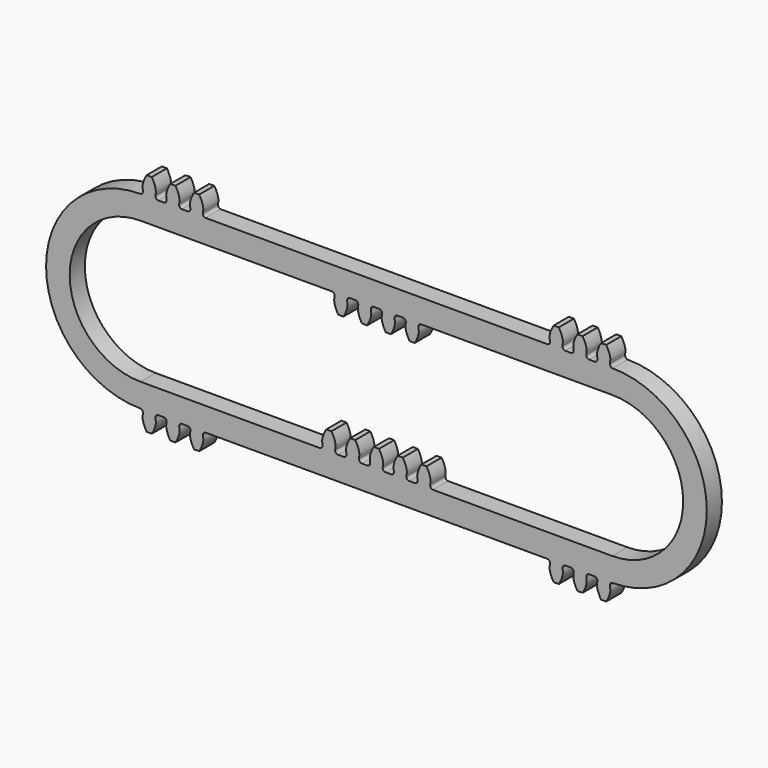
from build123d import *

# Parameters (mm, degrees)
F1_DEPTH = 5.08


# Not quite as in the source:
# - ends of sketch curves that miss each other by under 0.0002 mm in the source are joined
# - the dataset's text gives a spline's control points without its knots; the knots are read off the source's solid


with BuildPart() as f1:
    # F0 (on Front) → F1 (new body)
    with BuildSketch(Plane.XZ):
        with BuildLine():
            ThreePointArc((-63.3810963483, 25.3901347093), (-63.3753119036, 25.3901346444), (-63.3695274591, 25.3901332617))
            Line((-63.3695274591, 25.3901332617), (-58.7276592851, 25.3901332617))
            ThreePointArc((-58.7276592851, 25.3901332617), (-59.218266422, 25.7011127201), (-59.3684714986, 26.2622205719))
            add(Edge.make_bspline(
                [(-59.3684714986, 26.2622205719), (-59.31250661, 26.6931994762), (-59.2566199012, 27.1335892143), (-59.2570794401, 27.1878744736), (-59.2556284349, 27.2924728418), (-59.2623142438, 27.4188463575), (-59.2785741325, 27.5871922152), (-59.3088462635, 27.7897160279), (-59.3564984328, 28.027587018), (-59.4251457106, 28.298787), (-59.5181989128, 28.6019292415), (-59.6390373643, 28.9351012863), (-59.7906998965, 29.2962093017), (-59.9768979086, 29.6829308745), (-60.1697133275, 30.040270436), (-60.3087276421, 30.2685072323), (-60.3647969547, 30.359069462)],
                knots=[0.0609120431, 0.0609120431, 0.0609120431, 0.0609120431, 0.1648778545, 0.1947232852, 0.233253523, 0.2788430996, 0.3305368133, 0.38768636, 0.4498144648, 0.5165507531, 0.587596956, 0.6627061681, 0.7416696063, 0.8243077052, 0.9104638785, 0.9670212386, 0.9670212386, 0.9670212386, 0.9670212386], degree=3))
            Line((-60.3647969547, 30.359069462), (-61.7439586786, 30.359069462))
            add(Edge.make_bspline(
                [(-62.7402841346, 26.2622205719), (-62.7962490233, 26.6931994762), (-62.8521357321, 27.1335892143), (-62.8516761931, 27.1878744736), (-62.8531271984, 27.2924728418), (-62.8464413895, 27.4188463575), (-62.8301815007, 27.5871922152), (-62.7999093697, 27.7897160279), (-62.7522572004, 28.027587018), (-62.6836099226, 28.298787), (-62.5905567204, 28.6019292415), (-62.4697182689, 28.9351012863), (-62.3180557368, 29.2962093017), (-62.1318577246, 29.6829308745), (-61.9390423057, 30.040270436), (-61.8000279911, 30.2685072323), (-61.7439586786, 30.359069462)],
                knots=[0.0609120431, 0.0609120431, 0.0609120431, 0.0609120431, 0.1648778545, 0.1947232852, 0.233253523, 0.2788430996, 0.3305368133, 0.38768636, 0.4498144648, 0.5165507531, 0.587596956, 0.6627061681, 0.7416696063, 0.8243077052, 0.9104638785, 0.9670212386, 0.9670212386, 0.9670212386, 0.9670212386], degree=3))
            ThreePointArc((-62.7402841346, 26.2622205719), (-62.8904892112, 25.7011127201), (-63.3810963483, 25.3901347093))
        make_face()
        with BuildLine():
            Line((-58.7276592851, 25.3901332617), (-63.3695274591, 25.3901332617))
            ThreePointArc((-63.3695274591, 25.3901332617), (-63.3753119036, 25.3901346444), (-63.3810963483, 25.3901347093))
            ThreePointArc((-63.3810963483, 25.3901347093), (-88.7686237693, 0), (-63.3810963483, -25.3901347093))
            ThreePointArc((-63.3810963483, -25.3901347093), (-63.3753119036, -25.3901346444), (-63.3695274591, -25.3901332617))
            Line((-63.3695274591, -25.3901332617), (-58.7276592851, -25.3901332617))
            Line((-58.7276592851, -25.3901332617), (-57.0234432817, -25.3901332617))
            Line((-57.0234432817, -25.3901332617), (-52.3700062186, -25.3901332617))
            Line((-52.3700062186, -25.3901332617), (-50.6370496005, -25.3901332617))
            Line((-50.6370496005, -25.3901332617), (-45.9836125374, -25.3901332617))
            Line((-45.9836125374, -25.3901332617), (45.9836125374, -25.3901332617))
            Line((45.9836125374, -25.3901332617), (50.6370496005, -25.3901332617))
            Line((50.6370496005, -25.3901332617), (52.3700062186, -25.3901332617))
            Line((52.3700062186, -25.3901332617), (57.0234432817, -25.3901332617))
            Line((57.0234432817, -25.3901332617), (58.7276592851, -25.3901332617))
            Line((58.7276592851, -25.3901332617), (63.3695274591, -25.3901332617))
            ThreePointArc((63.3695274591, -25.3901332617), (63.3753119036, -25.3901346444), (63.3810963483, -25.3901347093))
            ThreePointArc((63.3810963483, -25.3901347093), (88.7686237693, 0), (63.3810963483, 25.3901347093))
            ThreePointArc((63.3810963483, 25.3901347093), (63.3753119036, 25.3901346444), (63.3695274591, 25.3901332617))
            Line((63.3695274591, 25.3901332617), (58.7276592851, 25.3901332617))
            Line((58.7276592851, 25.3901332617), (57.0234432817, 25.3901332617))
            Line((57.0234432817, 25.3901332617), (52.3700062186, 25.3901332617))
            Line((52.3700062186, 25.3901332617), (50.6370496005, 25.3901332617))
            Line((50.6370496005, 25.3901332617), (45.9836125374, 25.3901332617))
            Line((45.9836125374, 25.3901332617), (-45.9836125374, 25.3901332617))
            Line((-45.9836125374, 25.3901332617), (-50.6370496005, 25.3901332617))
            Line((-50.6370496005, 25.3901332617), (-52.3700062186, 25.3901332617))
            Line((-52.3700062186, 25.3901332617), (-57.0234432817, 25.3901332617))
            Line((-57.0234432817, 25.3901332617), (-58.7276592851, 25.3901332617))
        make_face()
        with BuildLine():
            ThreePointArc((-1.685906318, -18.1751586497), (-1.8361113946, -18.7362665015), (-2.3267185315, -19.0472459599))
            Line((-2.3267185315, -19.0472459599), (-4.0499982424, -19.0472459599))
            ThreePointArc((-4.0499982424, -19.0472459599), (-4.5406053793, -18.7362665015), (-4.6908104559, -18.1751586497))
            add(Edge.make_bspline(
                [(-4.6908104559, -18.1751586497), (-4.6348455673, -17.7441797454), (-4.5789588585, -17.3037900072), (-4.5794183974, -17.2495047479), (-4.5779673922, -17.1449063798), (-4.5846532011, -17.018532864), (-4.6009130899, -16.8501870063), (-4.6311852208, -16.6476631937), (-4.6788373902, -16.4097922035), (-4.747484668, -16.1385922215), (-4.8405378702, -15.8354499801), (-4.9613763217, -15.5022779353), (-5.1130388538, -15.1411699198), (-5.299236866, -14.754448347), (-5.4920522849, -14.3971087856), (-5.6310665994, -14.1688719893), (-5.687135912, -14.0783097595)],
                knots=[0.0609120431, 0.0609120431, 0.0609120431, 0.0609120431, 0.1648778545, 0.1947232852, 0.233253523, 0.2788430996, 0.3305368133, 0.38768636, 0.4498144648, 0.5165507531, 0.587596956, 0.6627061681, 0.7416696063, 0.8243077052, 0.9104638785, 0.9670212386, 0.9670212386, 0.9670212386, 0.9670212386], degree=3))
            Line((-5.687135912, -14.0783097595), (-6.376716774, -14.0783097595))
            Line((-6.376716774, -14.0783097595), (-7.0662976359, -14.0783097595))
            add(Edge.make_bspline(
                [(-8.062623092, -18.1751586497), (-8.1185879806, -17.7441797454), (-8.1744746894, -17.3037900072), (-8.1740151505, -17.2495047479), (-8.1754661557, -17.1449063798), (-8.1687803468, -17.018532864), (-8.1525204581, -16.8501870063), (-8.1222483271, -16.6476631937), (-8.0745961578, -16.4097922035), (-8.0059488799, -16.1385922215), (-7.9128956777, -15.8354499801), (-7.7920572263, -15.5022779353), (-7.6403946941, -15.1411699198), (-7.454196682, -14.754448347), (-7.261381263, -14.3971087856), (-7.1223669485, -14.1688719893), (-7.0662976359, -14.0783097595)],
                knots=[0.0609120431, 0.0609120431, 0.0609120431, 0.0609120431, 0.1648778545, 0.1947232852, 0.233253523, 0.2788430996, 0.3305368133, 0.38768636, 0.4498144648, 0.5165507531, 0.587596956, 0.6627061681, 0.7416696063, 0.8243077052, 0.9104638785, 0.9670212386, 0.9670212386, 0.9670212386, 0.9670212386], degree=3))
            ThreePointArc((-8.062623092, -18.1751586497), (-8.2128281686, -18.7362665015), (-8.7034353055, -19.0472459599))
            Line((-8.7034353055, -19.0472459599), (-10.4555296712, -19.0472459599))
            ThreePointArc((-10.4555296712, -19.0472459599), (-10.9461368081, -18.7362665015), (-11.0963418847, -18.1751586497))
            add(Edge.make_bspline(
                [(-11.0963418847, -18.1751586497), (-11.0403769961, -17.7441797454), (-10.9844902873, -17.3037900072), (-10.9849498262, -17.2495047479), (-10.983498821, -17.1449063798), (-10.9901846299, -17.018532864), (-11.0064445186, -16.8501870063), (-11.0367166496, -16.6476631937), (-11.0843688189, -16.4097922035), (-11.1530160967, -16.1385922215), (-11.2460692989, -15.8354499801), (-11.3669077504, -15.5022779353), (-11.5185702826, -15.1411699198), (-11.7047682947, -14.754448347), (-11.8975837136, -14.3971087856), (-12.0365980282, -14.1688719893), (-12.0926673408, -14.0783097595)],
                knots=[0.0609120431, 0.0609120431, 0.0609120431, 0.0609120431, 0.1648778545, 0.1947232852, 0.233253523, 0.2788430996, 0.3305368133, 0.38768636, 0.4498144648, 0.5165507531, 0.587596956, 0.6627061681, 0.7416696063, 0.8243077052, 0.9104638785, 0.9670212386, 0.9670212386, 0.9670212386, 0.9670212386], degree=3))
            Line((-12.0926673408, -14.0783097595), (-12.7822482027, -14.0783097595))
            Line((-12.7822482027, -14.0783097595), (-13.4718290647, -14.0783097595))
            add(Edge.make_bspline(
                [(-14.4681545207, -18.1751586497), (-14.5241194093, -17.7441797454), (-14.5800061182, -17.3037900072), (-14.5795465792, -17.2495047479), (-14.5809975845, -17.1449063798), (-14.5743117756, -17.018532864), (-14.5580518868, -16.8501870063), (-14.5277797558, -16.6476631937), (-14.4801275865, -16.4097922035), (-14.4114803087, -16.1385922215), (-14.3184271065, -15.8354499801), (-14.197588655, -15.5022779353), (-14.0459261229, -15.1411699198), (-13.8597281107, -14.754448347), (-13.6669126918, -14.3971087856), (-13.5278983772, -14.1688719893), (-13.4718290647, -14.0783097595)],
                knots=[0.0609120431, 0.0609120431, 0.0609120431, 0.0609120431, 0.1648778545, 0.1947232852, 0.233253523, 0.2788430996, 0.3305368133, 0.38768636, 0.4498144648, 0.5165507531, 0.587596956, 0.6627061681, 0.7416696063, 0.8243077052, 0.9104638785, 0.9670212386, 0.9670212386, 0.9670212386, 0.9670212386], degree=3))
            ThreePointArc((-14.4681545207, -18.1751586497), (-14.6183595973, -18.7362665015), (-15.1089667343, -19.0472459599))
            Line((-15.1089667343, -19.0472459599), (-63.3695274591, -19.0472459599))
            ThreePointArc((-63.3695274591, -19.0472459599), (-82.416773419, 0), (-63.3695274591, 19.0472459599))
            Line((-63.3695274591, 19.0472459599), (-11.8926318828, 19.0472459599))
            Line((-11.8926318828, 19.0472459599), (-7.2391948197, 19.0472459599))
            Line((-7.2391948197, 19.0472459599), (-5.517174257, 19.0472459599))
            Line((-5.517174257, 19.0472459599), (-0.8637371939, 19.0472459599))
            Line((-0.8637371939, 19.0472459599), (0.8637371939, 19.0472459599))
            Line((0.8637371939, 19.0472459599), (5.517174257, 19.0472459599))
            Line((5.517174257, 19.0472459599), (7.25960196, 19.0472459599))
            Line((7.25960196, 19.0472459599), (11.9130390231, 19.0472459599))
            Line((11.9130390231, 19.0472459599), (63.3695274591, 19.0472459599))
            ThreePointArc((63.3695274591, 19.0472459599), (82.416773419, 0), (63.3695274591, -19.0472459599))
            Line((63.3695274591, -19.0472459599), (15.0836943649, -19.0472459599))
            ThreePointArc((15.0836943649, -19.0472459599), (14.5930872279, -18.7362665015), (14.4428821513, -18.1751586497))
            add(Edge.make_bspline(
                [(14.4428821513, -18.1751586497), (14.49884704, -17.7441797454), (14.5547337488, -17.3037900072), (14.5542742099, -17.2495047479), (14.5557252151, -17.1449063798), (14.5490394062, -17.018532864), (14.5327795174, -16.8501870063), (14.5025073865, -16.6476631937), (14.4548552171, -16.4097922035), (14.3862079393, -16.1385922215), (14.2931547371, -15.8354499801), (14.1723162856, -15.5022779353), (14.0206537535, -15.1411699198), (13.8344557413, -14.754448347), (13.6416403224, -14.3971087856), (13.5026260079, -14.1688719893), (13.4465566953, -14.0783097595)],
                knots=[0.0609120431, 0.0609120431, 0.0609120431, 0.0609120431, 0.1648778545, 0.1947232852, 0.233253523, 0.2788430996, 0.3305368133, 0.38768636, 0.4498144648, 0.5165507531, 0.587596956, 0.6627061681, 0.7416696063, 0.8243077052, 0.9104638785, 0.9670212386, 0.9670212386, 0.9670212386, 0.9670212386], degree=3))
            Line((13.4465566953, -14.0783097595), (12.0673949714, -14.0783097595))
            add(Edge.make_bspline(
                [(11.0710695153, -18.1751586497), (11.0151046267, -17.7441797454), (10.9592179179, -17.3037900072), (10.9596774568, -17.2495047479), (10.9582264516, -17.1449063798), (10.9649122605, -17.018532864), (10.9811721492, -16.8501870063), (11.0114442802, -16.6476631937), (11.0590964495, -16.4097922035), (11.1277437273, -16.1385922215), (11.2207969295, -15.8354499801), (11.341635381, -15.5022779353), (11.4932979132, -15.1411699198), (11.6794959253, -14.754448347), (11.8723113443, -14.3971087856), (12.0113256588, -14.1688719893), (12.0673949714, -14.0783097595)],
                knots=[0.0609120431, 0.0609120431, 0.0609120431, 0.0609120431, 0.1648778545, 0.1947232852, 0.233253523, 0.2788430996, 0.3305368133, 0.38768636, 0.4498144648, 0.5165507531, 0.587596956, 0.6627061681, 0.7416696063, 0.8243077052, 0.9104638785, 0.9670212386, 0.9670212386, 0.9670212386, 0.9670212386], degree=3))
            ThreePointArc((11.0710695153, -18.1751586497), (10.9208644387, -18.7362665015), (10.4302573018, -19.0472459599))
            Line((10.4302573018, -19.0472459599), (8.7076299824, -19.0472459599))
            ThreePointArc((8.7076299824, -19.0472459599), (8.2170228455, -18.7362665015), (8.0668177688, -18.1751586497))
            add(Edge.make_bspline(
                [(8.0668177688, -18.1751586497), (8.1227826575, -17.7441797454), (8.1786693663, -17.3037900072), (8.1782098274, -17.2495047479), (8.1796608326, -17.1449063798), (8.1729750237, -17.018532864), (8.1567151349, -16.8501870063), (8.126443004, -16.6476631937), (8.0787908346, -16.4097922035), (8.0101435568, -16.1385922215), (7.9170903546, -15.8354499801), (7.7962519031, -15.5022779353), (7.644589371, -15.1411699198), (7.4583913588, -14.754448347), (7.2655759399, -14.3971087856), (7.1265616254, -14.1688719893), (7.0704923128, -14.0783097595)],
                knots=[0.0609120431, 0.0609120431, 0.0609120431, 0.0609120431, 0.1648778545, 0.1947232852, 0.233253523, 0.2788430996, 0.3305368133, 0.38768636, 0.4498144648, 0.5165507531, 0.587596956, 0.6627061681, 0.7416696063, 0.8243077052, 0.9104638785, 0.9670212386, 0.9670212386, 0.9670212386, 0.9670212386], degree=3))
            Line((7.0704923128, -14.0783097595), (5.6913305889, -14.0783097595))
            add(Edge.make_bspline(
                [(4.6950051328, -18.1751586497), (4.6390402442, -17.7441797454), (4.5831535354, -17.3037900072), (4.5836130743, -17.2495047479), (4.5821620691, -17.1449063798), (4.588847878, -17.018532864), (4.6051077667, -16.8501870063), (4.6353798977, -16.6476631937), (4.683032067, -16.4097922035), (4.7516793449, -16.1385922215), (4.844732547, -15.8354499801), (4.9655709985, -15.5022779353), (5.1172335307, -15.1411699198), (5.3034315428, -14.754448347), (5.4962469618, -14.3971087856), (5.6352612763, -14.1688719893), (5.6913305889, -14.0783097595)],
                knots=[0.0609120431, 0.0609120431, 0.0609120431, 0.0609120431, 0.1648778545, 0.1947232852, 0.233253523, 0.2788430996, 0.3305368133, 0.38768636, 0.4498144648, 0.5165507531, 0.587596956, 0.6627061681, 0.7416696063, 0.8243077052, 0.9104638785, 0.9670212386, 0.9670212386, 0.9670212386, 0.9670212386], degree=3))
            ThreePointArc((4.6950051328, -18.1751586497), (4.5448000562, -18.7362665015), (4.0541929193, -19.0472459599))
            Line((4.0541929193, -19.0472459599), (2.3267185315, -19.0472459599))
            ThreePointArc((2.3267185315, -19.0472459599), (1.8361113946, -18.7362665015), (1.685906318, -18.1751586497))
            add(Edge.make_bspline(
                [(1.685906318, -18.1751586497), (1.7418712066, -17.7441797454), (1.7977579155, -17.3037900072), (1.7972983765, -17.2495047479), (1.7987493818, -17.1449063798), (1.7920635729, -17.018532864), (1.7758036841, -16.8501870063), (1.7455315531, -16.6476631937), (1.6978793838, -16.4097922035), (1.629232106, -16.1385922215), (1.5361789038, -15.8354499801), (1.4153404523, -15.5022779353), (1.2636779201, -15.1411699198), (1.077479908, -14.754448347), (0.8846644891, -14.3971087856), (0.7456501745, -14.1688719893), (0.6895808619, -14.0783097595)],
                knots=[0.0609120431, 0.0609120431, 0.0609120431, 0.0609120431, 0.1648778545, 0.1947232852, 0.233253523, 0.2788430996, 0.3305368133, 0.38768636, 0.4498144648, 0.5165507531, 0.587596956, 0.6627061681, 0.7416696063, 0.8243077052, 0.9104638785, 0.9670212386, 0.9670212386, 0.9670212386, 0.9670212386], degree=3))
            Line((0.6895808619, -14.0783097595), (-0.6895808619, -14.0783097595))
            add(Edge.make_bspline(
                [(-1.685906318, -18.1751586497), (-1.7418712066, -17.7441797454), (-1.7977579155, -17.3037900072), (-1.7972983765, -17.2495047479), (-1.7987493818, -17.1449063798), (-1.7920635729, -17.018532864), (-1.7758036841, -16.8501870063), (-1.7455315531, -16.6476631937), (-1.6978793838, -16.4097922035), (-1.629232106, -16.1385922215), (-1.5361789038, -15.8354499801), (-1.4153404523, -15.5022779353), (-1.2636779201, -15.1411699198), (-1.077479908, -14.754448347), (-0.8846644891, -14.3971087856), (-0.7456501745, -14.1688719893), (-0.6895808619, -14.0783097595)],
                knots=[0.0609120431, 0.0609120431, 0.0609120431, 0.0609120431, 0.1648778545, 0.1947232852, 0.233253523, 0.2788430996, 0.3305368133, 0.38768636, 0.4498144648, 0.5165507531, 0.587596956, 0.6627061681, 0.7416696063, 0.8243077052, 0.9104638785, 0.9670212386, 0.9670212386, 0.9670212386, 0.9670212386], degree=3))
        make_face(mode=Mode.SUBTRACT)
        with BuildLine():
            ThreePointArc((-56.3826310681, 26.2622205719), (-56.5328361447, 25.7011127201), (-57.0234432817, 25.3901332617))
            Line((-57.0234432817, 25.3901332617), (-52.3700062186, 25.3901332617))
            ThreePointArc((-52.3700062186, 25.3901332617), (-52.8606133555, 25.7011127201), (-53.0108184321, 26.2622205719))
            add(Edge.make_bspline(
                [(-53.0108184321, 26.2622205719), (-52.9548535435, 26.6931994762), (-52.8989668346, 27.1335892143), (-52.8994263736, 27.1878744736), (-52.8979753683, 27.2924728418), (-52.9046611772, 27.4188463575), (-52.920921066, 27.5871922152), (-52.951193197, 27.7897160279), (-52.9988453663, 28.027587018), (-53.0674926441, 28.298787), (-53.1605458463, 28.6019292415), (-53.2813842978, 28.9351012863), (-53.43304683, 29.2962093017), (-53.6192448421, 29.6829308745), (-53.812060261, 30.040270436), (-53.9510745756, 30.2685072323), (-54.0071438882, 30.359069462)],
                knots=[0.0609120431, 0.0609120431, 0.0609120431, 0.0609120431, 0.1648778545, 0.1947232852, 0.233253523, 0.2788430996, 0.3305368133, 0.38768636, 0.4498144648, 0.5165507531, 0.587596956, 0.6627061681, 0.7416696063, 0.8243077052, 0.9104638785, 0.9670212386, 0.9670212386, 0.9670212386, 0.9670212386], degree=3))
            Line((-54.0071438882, 30.359069462), (-55.386305612, 30.359069462))
            add(Edge.make_bspline(
                [(-56.3826310681, 26.2622205719), (-56.4385959567, 26.6931994762), (-56.4944826656, 27.1335892143), (-56.4940231266, 27.1878744736), (-56.4954741319, 27.2924728418), (-56.488788323, 27.4188463575), (-56.4725284342, 27.5871922152), (-56.4422563032, 27.7897160279), (-56.3946041339, 28.027587018), (-56.3259568561, 28.298787), (-56.2329036539, 28.6019292415), (-56.1120652024, 28.9351012863), (-55.9604026702, 29.2962093017), (-55.7742046581, 29.6829308745), (-55.5813892392, 30.040270436), (-55.4423749246, 30.2685072323), (-55.386305612, 30.359069462)],
                knots=[0.0609120431, 0.0609120431, 0.0609120431, 0.0609120431, 0.1648778545, 0.1947232852, 0.233253523, 0.2788430996, 0.3305368133, 0.38768636, 0.4498144648, 0.5165507531, 0.587596956, 0.6627061681, 0.7416696063, 0.8243077052, 0.9104638785, 0.9670212386, 0.9670212386, 0.9670212386, 0.9670212386], degree=3))
        make_face()
        with BuildLine():
            ThreePointArc((-63.3695274591, -25.3901332617), (-63.3753119036, -25.3901346444), (-63.3810963483, -25.3901347093))
            ThreePointArc((-63.3810963483, -25.3901347093), (-62.8904892112, -25.7011127201), (-62.7402841346, -26.2622205719))
            add(Edge.make_bspline(
                [(-62.7402841346, -26.2622205719), (-62.7962490233, -26.6931994762), (-62.8521357321, -27.1335892143), (-62.8516761931, -27.1878744736), (-62.8531271984, -27.2924728418), (-62.8464413895, -27.4188463575), (-62.8301815007, -27.5871922152), (-62.7999093697, -27.7897160279), (-62.7522572004, -28.027587018), (-62.6836099226, -28.298787), (-62.5905567204, -28.6019292415), (-62.4697182689, -28.9351012863), (-62.3180557368, -29.2962093017), (-62.1318577246, -29.6829308745), (-61.9390423057, -30.040270436), (-61.8000279911, -30.2685072323), (-61.7439586786, -30.359069462)],
                knots=[0.0609120431, 0.0609120431, 0.0609120431, 0.0609120431, 0.1648778545, 0.1947232852, 0.233253523, 0.2788430996, 0.3305368133, 0.38768636, 0.4498144648, 0.5165507531, 0.587596956, 0.6627061681, 0.7416696063, 0.8243077052, 0.9104638785, 0.9670212386, 0.9670212386, 0.9670212386, 0.9670212386], degree=3))
            Line((-61.7439586786, -30.359069462), (-60.3647969547, -30.359069462))
            add(Edge.make_bspline(
                [(-59.3684714986, -26.2622205719), (-59.31250661, -26.6931994762), (-59.2566199012, -27.1335892143), (-59.2570794401, -27.1878744736), (-59.2556284349, -27.2924728418), (-59.2623142438, -27.4188463575), (-59.2785741325, -27.5871922152), (-59.3088462635, -27.7897160279), (-59.3564984328, -28.027587018), (-59.4251457106, -28.298787), (-59.5181989128, -28.6019292415), (-59.6390373643, -28.9351012863), (-59.7906998965, -29.2962093017), (-59.9768979086, -29.6829308745), (-60.1697133275, -30.040270436), (-60.3087276421, -30.2685072323), (-60.3647969547, -30.359069462)],
                knots=[0.0609120431, 0.0609120431, 0.0609120431, 0.0609120431, 0.1648778545, 0.1947232852, 0.233253523, 0.2788430996, 0.3305368133, 0.38768636, 0.4498144648, 0.5165507531, 0.587596956, 0.6627061681, 0.7416696063, 0.8243077052, 0.9104638785, 0.9670212386, 0.9670212386, 0.9670212386, 0.9670212386], degree=3))
            ThreePointArc((-59.3684714986, -26.2622205719), (-59.218266422, -25.7011127201), (-58.7276592851, -25.3901332617))
            Line((-58.7276592851, -25.3901332617), (-63.3695274591, -25.3901332617))
        make_face()
        with BuildLine():
            ThreePointArc((-49.9962373869, 26.2622205719), (-50.1464424636, 25.7011127201), (-50.6370496005, 25.3901332617))
            Line((-50.6370496005, 25.3901332617), (-45.9836125374, 25.3901332617))
            ThreePointArc((-45.9836125374, 25.3901332617), (-46.4742196743, 25.7011127201), (-46.6244247509, 26.2622205719))
            add(Edge.make_bspline(
                [(-46.6244247509, 26.2622205719), (-46.5684598623, 26.6931994762), (-46.5125731535, 27.1335892143), (-46.5130326924, 27.1878744736), (-46.5115816872, 27.2924728418), (-46.5182674961, 27.4188463575), (-46.5345273848, 27.5871922152), (-46.5647995158, 27.7897160279), (-46.6124516851, 28.027587018), (-46.681098963, 28.298787), (-46.7741521651, 28.6019292415), (-46.8949906166, 28.9351012863), (-47.0466531488, 29.2962093017), (-47.2328511609, 29.6829308745), (-47.4256665799, 30.040270436), (-47.5646808944, 30.2685072323), (-47.620750207, 30.359069462)],
                knots=[0.0609120431, 0.0609120431, 0.0609120431, 0.0609120431, 0.1648778545, 0.1947232852, 0.233253523, 0.2788430996, 0.3305368133, 0.38768636, 0.4498144648, 0.5165507531, 0.587596956, 0.6627061681, 0.7416696063, 0.8243077052, 0.9104638785, 0.9670212386, 0.9670212386, 0.9670212386, 0.9670212386], degree=3))
            Line((-47.620750207, 30.359069462), (-48.9999119309, 30.359069462))
            add(Edge.make_bspline(
                [(-49.9962373869, 26.2622205719), (-50.0522022756, 26.6931994762), (-50.1080889844, 27.1335892143), (-50.1076294455, 27.1878744736), (-50.1090804507, 27.2924728418), (-50.1023946418, 27.4188463575), (-50.086134753, 27.5871922152), (-50.0558626221, 27.7897160279), (-50.0082104527, 28.027587018), (-49.9395631749, 28.298787), (-49.8465099727, 28.6019292415), (-49.7256715212, 28.9351012863), (-49.5740089891, 29.2962093017), (-49.3878109769, 29.6829308745), (-49.194995558, 30.040270436), (-49.0559812435, 30.2685072323), (-48.9999119309, 30.359069462)],
                knots=[0.0609120431, 0.0609120431, 0.0609120431, 0.0609120431, 0.1648778545, 0.1947232852, 0.233253523, 0.2788430996, 0.3305368133, 0.38768636, 0.4498144648, 0.5165507531, 0.587596956, 0.6627061681, 0.7416696063, 0.8243077052, 0.9104638785, 0.9670212386, 0.9670212386, 0.9670212386, 0.9670212386], degree=3))
        make_face()
        with BuildLine():
            Line((-52.3700062186, -25.3901332617), (-57.0234432817, -25.3901332617))
            ThreePointArc((-57.0234432817, -25.3901332617), (-56.5328361447, -25.7011127201), (-56.3826310681, -26.2622205719))
            add(Edge.make_bspline(
                [(-56.3826310681, -26.2622205719), (-56.4385959567, -26.6931994762), (-56.4944826656, -27.1335892143), (-56.4940231266, -27.1878744736), (-56.4954741319, -27.2924728418), (-56.488788323, -27.4188463575), (-56.4725284342, -27.5871922152), (-56.4422563032, -27.7897160279), (-56.3946041339, -28.027587018), (-56.3259568561, -28.298787), (-56.2329036539, -28.6019292415), (-56.1120652024, -28.9351012863), (-55.9604026702, -29.2962093017), (-55.7742046581, -29.6829308745), (-55.5813892392, -30.040270436), (-55.4423749246, -30.2685072323), (-55.386305612, -30.359069462)],
                knots=[0.0609120431, 0.0609120431, 0.0609120431, 0.0609120431, 0.1648778545, 0.1947232852, 0.233253523, 0.2788430996, 0.3305368133, 0.38768636, 0.4498144648, 0.5165507531, 0.587596956, 0.6627061681, 0.7416696063, 0.8243077052, 0.9104638785, 0.9670212386, 0.9670212386, 0.9670212386, 0.9670212386], degree=3))
            Line((-55.386305612, -30.359069462), (-54.0071438882, -30.359069462))
            add(Edge.make_bspline(
                [(-53.0108184321, -26.2622205719), (-52.9548535435, -26.6931994762), (-52.8989668346, -27.1335892143), (-52.8994263736, -27.1878744736), (-52.8979753683, -27.2924728418), (-52.9046611772, -27.4188463575), (-52.920921066, -27.5871922152), (-52.951193197, -27.7897160279), (-52.9988453663, -28.027587018), (-53.0674926441, -28.298787), (-53.1605458463, -28.6019292415), (-53.2813842978, -28.9351012863), (-53.43304683, -29.2962093017), (-53.6192448421, -29.6829308745), (-53.812060261, -30.040270436), (-53.9510745756, -30.2685072323), (-54.0071438882, -30.359069462)],
                knots=[0.0609120431, 0.0609120431, 0.0609120431, 0.0609120431, 0.1648778545, 0.1947232852, 0.233253523, 0.2788430996, 0.3305368133, 0.38768636, 0.4498144648, 0.5165507531, 0.587596956, 0.6627061681, 0.7416696063, 0.8243077052, 0.9104638785, 0.9670212386, 0.9670212386, 0.9670212386, 0.9670212386], degree=3))
            ThreePointArc((-53.0108184321, -26.2622205719), (-52.8606133555, -25.7011127201), (-52.3700062186, -25.3901332617))
        make_face()
        with BuildLine():
            ThreePointArc((46.6244247509, 26.2622205719), (46.4742196743, 25.7011127201), (45.9836125374, 25.3901332617))
            Line((45.9836125374, 25.3901332617), (50.6370496005, 25.3901332617))
            ThreePointArc((50.6370496005, 25.3901332617), (50.1464424636, 25.7011127201), (49.9962373869, 26.2622205719))
            add(Edge.make_bspline(
                [(49.9962373869, 26.2622205719), (50.0522022756, 26.6931994762), (50.1080889844, 27.1335892143), (50.1076294455, 27.1878744736), (50.1090804507, 27.2924728418), (50.1023946418, 27.4188463575), (50.086134753, 27.5871922152), (50.0558626221, 27.7897160279), (50.0082104527, 28.027587018), (49.9395631749, 28.298787), (49.8465099727, 28.6019292415), (49.7256715212, 28.9351012863), (49.5740089891, 29.2962093017), (49.3878109769, 29.6829308745), (49.194995558, 30.040270436), (49.0559812435, 30.2685072323), (48.9999119309, 30.359069462)],
                knots=[0.0609120431, 0.0609120431, 0.0609120431, 0.0609120431, 0.1648778545, 0.1947232852, 0.233253523, 0.2788430996, 0.3305368133, 0.38768636, 0.4498144648, 0.5165507531, 0.587596956, 0.6627061681, 0.7416696063, 0.8243077052, 0.9104638785, 0.9670212386, 0.9670212386, 0.9670212386, 0.9670212386], degree=3))
            Line((48.9999119309, 30.359069462), (47.620750207, 30.359069462))
            add(Edge.make_bspline(
                [(46.6244247509, 26.2622205719), (46.5684598623, 26.6931994762), (46.5125731535, 27.1335892143), (46.5130326924, 27.1878744736), (46.5115816872, 27.2924728418), (46.5182674961, 27.4188463575), (46.5345273848, 27.5871922152), (46.5647995158, 27.7897160279), (46.6124516851, 28.027587018), (46.681098963, 28.298787), (46.7741521651, 28.6019292415), (46.8949906166, 28.9351012863), (47.0466531488, 29.2962093017), (47.2328511609, 29.6829308745), (47.4256665799, 30.040270436), (47.5646808944, 30.2685072323), (47.620750207, 30.359069462)],
                knots=[0.0609120431, 0.0609120431, 0.0609120431, 0.0609120431, 0.1648778545, 0.1947232852, 0.233253523, 0.2788430996, 0.3305368133, 0.38768636, 0.4498144648, 0.5165507531, 0.587596956, 0.6627061681, 0.7416696063, 0.8243077052, 0.9104638785, 0.9670212386, 0.9670212386, 0.9670212386, 0.9670212386], degree=3))
        make_face()
        with BuildLine():
            Line((-45.9836125374, -25.3901332617), (-50.6370496005, -25.3901332617))
            ThreePointArc((-50.6370496005, -25.3901332617), (-50.1464424636, -25.7011127201), (-49.9962373869, -26.2622205719))
            add(Edge.make_bspline(
                [(-49.9962373869, -26.2622205719), (-50.0522022756, -26.6931994762), (-50.1080889844, -27.1335892143), (-50.1076294455, -27.1878744736), (-50.1090804507, -27.2924728418), (-50.1023946418, -27.4188463575), (-50.086134753, -27.5871922152), (-50.0558626221, -27.7897160279), (-50.0082104527, -28.027587018), (-49.9395631749, -28.298787), (-49.8465099727, -28.6019292415), (-49.7256715212, -28.9351012863), (-49.5740089891, -29.2962093017), (-49.3878109769, -29.6829308745), (-49.194995558, -30.040270436), (-49.0559812435, -30.2685072323), (-48.9999119309, -30.359069462)],
                knots=[0.0609120431, 0.0609120431, 0.0609120431, 0.0609120431, 0.1648778545, 0.1947232852, 0.233253523, 0.2788430996, 0.3305368133, 0.38768636, 0.4498144648, 0.5165507531, 0.587596956, 0.6627061681, 0.7416696063, 0.8243077052, 0.9104638785, 0.9670212386, 0.9670212386, 0.9670212386, 0.9670212386], degree=3))
            Line((-48.9999119309, -30.359069462), (-47.620750207, -30.359069462))
            add(Edge.make_bspline(
                [(-46.6244247509, -26.2622205719), (-46.5684598623, -26.6931994762), (-46.5125731535, -27.1335892143), (-46.5130326924, -27.1878744736), (-46.5115816872, -27.2924728418), (-46.5182674961, -27.4188463575), (-46.5345273848, -27.5871922152), (-46.5647995158, -27.7897160279), (-46.6124516851, -28.027587018), (-46.681098963, -28.298787), (-46.7741521651, -28.6019292415), (-46.8949906166, -28.9351012863), (-47.0466531488, -29.2962093017), (-47.2328511609, -29.6829308745), (-47.4256665799, -30.040270436), (-47.5646808944, -30.2685072323), (-47.620750207, -30.359069462)],
                knots=[0.0609120431, 0.0609120431, 0.0609120431, 0.0609120431, 0.1648778545, 0.1947232852, 0.233253523, 0.2788430996, 0.3305368133, 0.38768636, 0.4498144648, 0.5165507531, 0.587596956, 0.6627061681, 0.7416696063, 0.8243077052, 0.9104638785, 0.9670212386, 0.9670212386, 0.9670212386, 0.9670212386], degree=3))
            ThreePointArc((-46.6244247509, -26.2622205719), (-46.4742196743, -25.7011127201), (-45.9836125374, -25.3901332617))
        make_face()
        with BuildLine():
            ThreePointArc((53.0108184321, 26.2622205719), (52.8606133555, 25.7011127201), (52.3700062186, 25.3901332617))
            Line((52.3700062186, 25.3901332617), (57.0234432817, 25.3901332617))
            ThreePointArc((57.0234432817, 25.3901332617), (56.5328361447, 25.7011127201), (56.3826310681, 26.2622205719))
            add(Edge.make_bspline(
                [(56.3826310681, 26.2622205719), (56.4385959567, 26.6931994762), (56.4944826656, 27.1335892143), (56.4940231266, 27.1878744736), (56.4954741319, 27.2924728418), (56.488788323, 27.4188463575), (56.4725284342, 27.5871922152), (56.4422563032, 27.7897160279), (56.3946041339, 28.027587018), (56.3259568561, 28.298787), (56.2329036539, 28.6019292415), (56.1120652024, 28.9351012863), (55.9604026702, 29.2962093017), (55.7742046581, 29.6829308745), (55.5813892392, 30.040270436), (55.4423749246, 30.2685072323), (55.386305612, 30.359069462)],
                knots=[0.0609120431, 0.0609120431, 0.0609120431, 0.0609120431, 0.1648778545, 0.1947232852, 0.233253523, 0.2788430996, 0.3305368133, 0.38768636, 0.4498144648, 0.5165507531, 0.587596956, 0.6627061681, 0.7416696063, 0.8243077052, 0.9104638785, 0.9670212386, 0.9670212386, 0.9670212386, 0.9670212386], degree=3))
            Line((55.386305612, 30.359069462), (54.0071438882, 30.359069462))
            add(Edge.make_bspline(
                [(53.0108184321, 26.2622205719), (52.9548535435, 26.6931994762), (52.8989668346, 27.1335892143), (52.8994263736, 27.1878744736), (52.8979753683, 27.2924728418), (52.9046611772, 27.4188463575), (52.920921066, 27.5871922152), (52.951193197, 27.7897160279), (52.9988453663, 28.027587018), (53.0674926441, 28.298787), (53.1605458463, 28.6019292415), (53.2813842978, 28.9351012863), (53.43304683, 29.2962093017), (53.6192448421, 29.6829308745), (53.812060261, 30.040270436), (53.9510745756, 30.2685072323), (54.0071438882, 30.359069462)],
                knots=[0.0609120431, 0.0609120431, 0.0609120431, 0.0609120431, 0.1648778545, 0.1947232852, 0.233253523, 0.2788430996, 0.3305368133, 0.38768636, 0.4498144648, 0.5165507531, 0.587596956, 0.6627061681, 0.7416696063, 0.8243077052, 0.9104638785, 0.9670212386, 0.9670212386, 0.9670212386, 0.9670212386], degree=3))
        make_face()
        with BuildLine():
            Line((50.6370496005, -25.3901332617), (45.9836125374, -25.3901332617))
            ThreePointArc((45.9836125374, -25.3901332617), (46.4742196743, -25.7011127201), (46.6244247509, -26.2622205719))
            add(Edge.make_bspline(
                [(46.6244247509, -26.2622205719), (46.5684598623, -26.6931994762), (46.5125731535, -27.1335892143), (46.5130326924, -27.1878744736), (46.5115816872, -27.2924728418), (46.5182674961, -27.4188463575), (46.5345273848, -27.5871922152), (46.5647995158, -27.7897160279), (46.6124516851, -28.027587018), (46.681098963, -28.298787), (46.7741521651, -28.6019292415), (46.8949906166, -28.9351012863), (47.0466531488, -29.2962093017), (47.2328511609, -29.6829308745), (47.4256665799, -30.040270436), (47.5646808944, -30.2685072323), (47.620750207, -30.359069462)],
                knots=[0.0609120431, 0.0609120431, 0.0609120431, 0.0609120431, 0.1648778545, 0.1947232852, 0.233253523, 0.2788430996, 0.3305368133, 0.38768636, 0.4498144648, 0.5165507531, 0.587596956, 0.6627061681, 0.7416696063, 0.8243077052, 0.9104638785, 0.9670212386, 0.9670212386, 0.9670212386, 0.9670212386], degree=3))
            Line((47.620750207, -30.359069462), (48.9999119309, -30.359069462))
            add(Edge.make_bspline(
                [(49.9962373869, -26.2622205719), (50.0522022756, -26.6931994762), (50.1080889844, -27.1335892143), (50.1076294455, -27.1878744736), (50.1090804507, -27.2924728418), (50.1023946418, -27.4188463575), (50.086134753, -27.5871922152), (50.0558626221, -27.7897160279), (50.0082104527, -28.027587018), (49.9395631749, -28.298787), (49.8465099727, -28.6019292415), (49.7256715212, -28.9351012863), (49.5740089891, -29.2962093017), (49.3878109769, -29.6829308745), (49.194995558, -30.040270436), (49.0559812435, -30.2685072323), (48.9999119309, -30.359069462)],
                knots=[0.0609120431, 0.0609120431, 0.0609120431, 0.0609120431, 0.1648778545, 0.1947232852, 0.233253523, 0.2788430996, 0.3305368133, 0.38768636, 0.4498144648, 0.5165507531, 0.587596956, 0.6627061681, 0.7416696063, 0.8243077052, 0.9104638785, 0.9670212386, 0.9670212386, 0.9670212386, 0.9670212386], degree=3))
            ThreePointArc((49.9962373869, -26.2622205719), (50.1464424636, -25.7011127201), (50.6370496005, -25.3901332617))
        make_face()
        with BuildLine():
            ThreePointArc((59.3684714986, 26.2622205719), (59.218266422, 25.7011127201), (58.7276592851, 25.3901332617))
            Line((58.7276592851, 25.3901332617), (63.3695274591, 25.3901332617))
            ThreePointArc((63.3695274591, 25.3901332617), (63.3753119036, 25.3901346444), (63.3810963483, 25.3901347093))
            ThreePointArc((63.3810963483, 25.3901347093), (62.8904892112, 25.7011127201), (62.7402841346, 26.2622205719))
            add(Edge.make_bspline(
                [(62.7402841346, 26.2622205719), (62.7962490233, 26.6931994762), (62.8521357321, 27.1335892143), (62.8516761931, 27.1878744736), (62.8531271984, 27.2924728418), (62.8464413895, 27.4188463575), (62.8301815007, 27.5871922152), (62.7999093697, 27.7897160279), (62.7522572004, 28.027587018), (62.6836099226, 28.298787), (62.5905567204, 28.6019292415), (62.4697182689, 28.9351012863), (62.3180557368, 29.2962093017), (62.1318577246, 29.6829308745), (61.9390423057, 30.040270436), (61.8000279911, 30.2685072323), (61.7439586786, 30.359069462)],
                knots=[0.0609120431, 0.0609120431, 0.0609120431, 0.0609120431, 0.1648778545, 0.1947232852, 0.233253523, 0.2788430996, 0.3305368133, 0.38768636, 0.4498144648, 0.5165507531, 0.587596956, 0.6627061681, 0.7416696063, 0.8243077052, 0.9104638785, 0.9670212386, 0.9670212386, 0.9670212386, 0.9670212386], degree=3))
            Line((61.7439586786, 30.359069462), (60.3647969547, 30.359069462))
            add(Edge.make_bspline(
                [(59.3684714986, 26.2622205719), (59.31250661, 26.6931994762), (59.2566199012, 27.1335892143), (59.2570794401, 27.1878744736), (59.2556284349, 27.2924728418), (59.2623142438, 27.4188463575), (59.2785741325, 27.5871922152), (59.3088462635, 27.7897160279), (59.3564984328, 28.027587018), (59.4251457106, 28.298787), (59.5181989128, 28.6019292415), (59.6390373643, 28.9351012863), (59.7906998965, 29.2962093017), (59.9768979086, 29.6829308745), (60.1697133275, 30.040270436), (60.3087276421, 30.2685072323), (60.3647969547, 30.359069462)],
                knots=[0.0609120431, 0.0609120431, 0.0609120431, 0.0609120431, 0.1648778545, 0.1947232852, 0.233253523, 0.2788430996, 0.3305368133, 0.38768636, 0.4498144648, 0.5165507531, 0.587596956, 0.6627061681, 0.7416696063, 0.8243077052, 0.9104638785, 0.9670212386, 0.9670212386, 0.9670212386, 0.9670212386], degree=3))
        make_face()
        with BuildLine():
            Line((57.0234432817, -25.3901332617), (52.3700062186, -25.3901332617))
            ThreePointArc((52.3700062186, -25.3901332617), (52.8606133555, -25.7011127201), (53.0108184321, -26.2622205719))
            add(Edge.make_bspline(
                [(53.0108184321, -26.2622205719), (52.9548535435, -26.6931994762), (52.8989668346, -27.1335892143), (52.8994263736, -27.1878744736), (52.8979753683, -27.2924728418), (52.9046611772, -27.4188463575), (52.920921066, -27.5871922152), (52.951193197, -27.7897160279), (52.9988453663, -28.027587018), (53.0674926441, -28.298787), (53.1605458463, -28.6019292415), (53.2813842978, -28.9351012863), (53.43304683, -29.2962093017), (53.6192448421, -29.6829308745), (53.812060261, -30.040270436), (53.9510745756, -30.2685072323), (54.0071438882, -30.359069462)],
                knots=[0.0609120431, 0.0609120431, 0.0609120431, 0.0609120431, 0.1648778545, 0.1947232852, 0.233253523, 0.2788430996, 0.3305368133, 0.38768636, 0.4498144648, 0.5165507531, 0.587596956, 0.6627061681, 0.7416696063, 0.8243077052, 0.9104638785, 0.9670212386, 0.9670212386, 0.9670212386, 0.9670212386], degree=3))
            Line((54.0071438882, -30.359069462), (55.386305612, -30.359069462))
            add(Edge.make_bspline(
                [(56.3826310681, -26.2622205719), (56.4385959567, -26.6931994762), (56.4944826656, -27.1335892143), (56.4940231266, -27.1878744736), (56.4954741319, -27.2924728418), (56.488788323, -27.4188463575), (56.4725284342, -27.5871922152), (56.4422563032, -27.7897160279), (56.3946041339, -28.027587018), (56.3259568561, -28.298787), (56.2329036539, -28.6019292415), (56.1120652024, -28.9351012863), (55.9604026702, -29.2962093017), (55.7742046581, -29.6829308745), (55.5813892392, -30.040270436), (55.4423749246, -30.2685072323), (55.386305612, -30.359069462)],
                knots=[0.0609120431, 0.0609120431, 0.0609120431, 0.0609120431, 0.1648778545, 0.1947232852, 0.233253523, 0.2788430996, 0.3305368133, 0.38768636, 0.4498144648, 0.5165507531, 0.587596956, 0.6627061681, 0.7416696063, 0.8243077052, 0.9104638785, 0.9670212386, 0.9670212386, 0.9670212386, 0.9670212386], degree=3))
            ThreePointArc((56.3826310681, -26.2622205719), (56.5328361447, -25.7011127201), (57.0234432817, -25.3901332617))
        make_face()
        with BuildLine():
            ThreePointArc((62.7402841346, -26.2622205719), (62.8904892112, -25.7011127201), (63.3810963482, -25.3901332617))
            ThreePointArc((63.3810963482, -25.3901332617), (63.3753119036, -25.3901346444), (63.3695274591, -25.3901332617))
            Line((63.3695274591, -25.3901332617), (58.7276592851, -25.3901332617))
            ThreePointArc((58.7276592851, -25.3901332617), (59.218266422, -25.7011127201), (59.3684714986, -26.2622205719))
            add(Edge.make_bspline(
                [(59.3684714986, -26.2622205719), (59.31250661, -26.6931994762), (59.2566199012, -27.1335892143), (59.2570794401, -27.1878744736), (59.2556284349, -27.2924728418), (59.2623142438, -27.4188463575), (59.2785741325, -27.5871922152), (59.3088462635, -27.7897160279), (59.3564984328, -28.027587018), (59.4251457106, -28.298787), (59.5181989128, -28.6019292415), (59.6390373643, -28.9351012863), (59.7906998965, -29.2962093017), (59.9768979086, -29.6829308745), (60.1697133275, -30.040270436), (60.3087276421, -30.2685072323), (60.3647969547, -30.359069462)],
                knots=[0.0609120431, 0.0609120431, 0.0609120431, 0.0609120431, 0.1648778545, 0.1947232852, 0.233253523, 0.2788430996, 0.3305368133, 0.38768636, 0.4498144648, 0.5165507531, 0.587596956, 0.6627061681, 0.7416696063, 0.8243077052, 0.9104638785, 0.9670212386, 0.9670212386, 0.9670212386, 0.9670212386], degree=3))
            Line((60.3647969547, -30.359069462), (61.7439586786, -30.359069462))
            add(Edge.make_bspline(
                [(62.7402841346, -26.2622205719), (62.7962490233, -26.6931994762), (62.8521357321, -27.1335892143), (62.8516761931, -27.1878744736), (62.8531271984, -27.2924728418), (62.8464413895, -27.4188463575), (62.8301815007, -27.5871922152), (62.7999093697, -27.7897160279), (62.7522572004, -28.027587018), (62.6836099226, -28.298787), (62.5905567204, -28.6019292415), (62.4697182689, -28.9351012863), (62.3180557368, -29.2962093017), (62.1318577246, -29.6829308745), (61.9390423057, -30.040270436), (61.8000279911, -30.2685072323), (61.7439586786, -30.359069462)],
                knots=[0.0609120431, 0.0609120431, 0.0609120431, 0.0609120431, 0.1648778545, 0.1947232852, 0.233253523, 0.2788430996, 0.3305368133, 0.38768636, 0.4498144648, 0.5165507531, 0.587596956, 0.6627061681, 0.7416696063, 0.8243077052, 0.9104638785, 0.9670212386, 0.9670212386, 0.9670212386, 0.9670212386], degree=3))
        make_face()
        with BuildLine():
            Line((-7.2391948197, 19.0472459599), (-11.8926318828, 19.0472459599))
            ThreePointArc((-11.8926318828, 19.0472459599), (-11.4020247459, 18.7362665015), (-11.2518196693, 18.1751586497))
            add(Edge.make_bspline(
                [(-11.2518196693, 18.1751586497), (-11.3077845579, 17.7441797454), (-11.3636712667, 17.3037900072), (-11.3632117278, 17.2495047479), (-11.364662733, 17.1449063798), (-11.3579769241, 17.018532864), (-11.3417170354, 16.8501870063), (-11.3114449044, 16.6476631937), (-11.2637927351, 16.4097922035), (-11.1951454572, 16.1385922215), (-11.102092255, 15.8354499801), (-10.9812538035, 15.5022779353), (-10.8295912714, 15.1411699198), (-10.6433932593, 14.754448347), (-10.4505778403, 14.3971087856), (-10.3115635258, 14.1688719893), (-10.2554942132, 14.0783097595)],
                knots=[0.0609120431, 0.0609120431, 0.0609120431, 0.0609120431, 0.1648778545, 0.1947232852, 0.233253523, 0.2788430996, 0.3305368133, 0.38768636, 0.4498144648, 0.5165507531, 0.587596956, 0.6627061681, 0.7416696063, 0.8243077052, 0.9104638785, 0.9670212386, 0.9670212386, 0.9670212386, 0.9670212386], degree=3))
            Line((-10.2554942132, 14.0783097595), (-8.8763324893, 14.0783097595))
            add(Edge.make_bspline(
                [(-7.8800070332, 18.1751586497), (-7.8240421446, 17.7441797454), (-7.7681554358, 17.3037900072), (-7.7686149747, 17.2495047479), (-7.7671639695, 17.1449063798), (-7.7738497784, 17.018532864), (-7.7901096671, 16.8501870063), (-7.8203817981, 16.6476631937), (-7.8680339675, 16.4097922035), (-7.9366812453, 16.1385922215), (-8.0297344475, 15.8354499801), (-8.150572899, 15.5022779353), (-8.3022354311, 15.1411699198), (-8.4884334432, 14.754448347), (-8.6812488622, 14.3971087856), (-8.8202631767, 14.1688719893), (-8.8763324893, 14.0783097595)],
                knots=[0.0609120431, 0.0609120431, 0.0609120431, 0.0609120431, 0.1648778545, 0.1947232852, 0.233253523, 0.2788430996, 0.3305368133, 0.38768636, 0.4498144648, 0.5165507531, 0.587596956, 0.6627061681, 0.7416696063, 0.8243077052, 0.9104638785, 0.9670212386, 0.9670212386, 0.9670212386, 0.9670212386], degree=3))
            ThreePointArc((-7.8800070332, 18.1751586497), (-7.7298019566, 18.7362665015), (-7.2391948197, 19.0472459599))
        make_face()
        with BuildLine():
            Line((-0.8637371939, 19.0472459599), (-5.517174257, 19.0472459599))
            ThreePointArc((-5.517174257, 19.0472459599), (-5.02656712, 18.7362665015), (-4.8763620434, 18.1751586497))
            add(Edge.make_bspline(
                [(-4.8763620434, 18.1751586497), (-4.9323269321, 17.7441797454), (-4.9882136409, 17.3037900072), (-4.9877541019, 17.2495047479), (-4.9892051072, 17.1449063798), (-4.9825192983, 17.018532864), (-4.9662594095, 16.8501870063), (-4.9359872785, 16.6476631937), (-4.8883351092, 16.4097922035), (-4.8196878314, 16.1385922215), (-4.7266346292, 15.8354499801), (-4.6057961777, 15.5022779353), (-4.4541336456, 15.1411699198), (-4.2679356334, 14.754448347), (-4.0751202145, 14.3971087856), (-3.9361058999, 14.1688719893), (-3.8800365874, 14.0783097595)],
                knots=[0.0609120431, 0.0609120431, 0.0609120431, 0.0609120431, 0.1648778545, 0.1947232852, 0.233253523, 0.2788430996, 0.3305368133, 0.38768636, 0.4498144648, 0.5165507531, 0.587596956, 0.6627061681, 0.7416696063, 0.8243077052, 0.9104638785, 0.9670212386, 0.9670212386, 0.9670212386, 0.9670212386], degree=3))
            Line((-3.8800365874, 14.0783097595), (-2.5008748635, 14.0783097595))
            add(Edge.make_bspline(
                [(-1.5045494074, 18.1751586497), (-1.4485845188, 17.7441797454), (-1.39269781, 17.3037900072), (-1.3931573489, 17.2495047479), (-1.3917063437, 17.1449063798), (-1.3983921526, 17.018532864), (-1.4146520413, 16.8501870063), (-1.4449241723, 16.6476631937), (-1.4925763416, 16.4097922035), (-1.5612236194, 16.1385922215), (-1.6542768216, 15.8354499801), (-1.7751152731, 15.5022779353), (-1.9267778053, 15.1411699198), (-2.1129758174, 14.754448347), (-2.3057912363, 14.3971087856), (-2.4448055509, 14.1688719893), (-2.5008748635, 14.0783097595)],
                knots=[0.0609120431, 0.0609120431, 0.0609120431, 0.0609120431, 0.1648778545, 0.1947232852, 0.233253523, 0.2788430996, 0.3305368133, 0.38768636, 0.4498144648, 0.5165507531, 0.587596956, 0.6627061681, 0.7416696063, 0.8243077052, 0.9104638785, 0.9670212386, 0.9670212386, 0.9670212386, 0.9670212386], degree=3))
            ThreePointArc((-1.5045494074, 18.1751586497), (-1.3543443308, 18.7362665015), (-0.8637371939, 19.0472459599))
        make_face()
        with BuildLine():
            Line((5.517174257, 19.0472459599), (0.8637371939, 19.0472459599))
            ThreePointArc((0.8637371939, 19.0472459599), (1.3543443308, 18.7362665015), (1.5045494074, 18.1751586497))
            add(Edge.make_bspline(
                [(1.5045494074, 18.1751586497), (1.4485845188, 17.7441797454), (1.39269781, 17.3037900072), (1.3931573489, 17.2495047479), (1.3917063437, 17.1449063798), (1.3983921526, 17.018532864), (1.4146520413, 16.8501870063), (1.4449241723, 16.6476631937), (1.4925763416, 16.4097922035), (1.5612236194, 16.1385922215), (1.6542768216, 15.8354499801), (1.7751152731, 15.5022779353), (1.9267778053, 15.1411699198), (2.1129758174, 14.754448347), (2.3057912363, 14.3971087856), (2.4448055509, 14.1688719893), (2.5008748635, 14.0783097595)],
                knots=[0.0609120431, 0.0609120431, 0.0609120431, 0.0609120431, 0.1648778545, 0.1947232852, 0.233253523, 0.2788430996, 0.3305368133, 0.38768636, 0.4498144648, 0.5165507531, 0.587596956, 0.6627061681, 0.7416696063, 0.8243077052, 0.9104638785, 0.9670212386, 0.9670212386, 0.9670212386, 0.9670212386], degree=3))
            Line((2.5008748635, 14.0783097595), (3.8800365874, 14.0783097595))
            add(Edge.make_bspline(
                [(4.8763620434, 18.1751586497), (4.9323269321, 17.7441797454), (4.9882136409, 17.3037900072), (4.9877541019, 17.2495047479), (4.9892051072, 17.1449063798), (4.9825192983, 17.018532864), (4.9662594095, 16.8501870063), (4.9359872785, 16.6476631937), (4.8883351092, 16.4097922035), (4.8196878314, 16.1385922215), (4.7266346292, 15.8354499801), (4.6057961777, 15.5022779353), (4.4541336456, 15.1411699198), (4.2679356334, 14.754448347), (4.0751202145, 14.3971087856), (3.9361058999, 14.1688719893), (3.8800365874, 14.0783097595)],
                knots=[0.0609120431, 0.0609120431, 0.0609120431, 0.0609120431, 0.1648778545, 0.1947232852, 0.233253523, 0.2788430996, 0.3305368133, 0.38768636, 0.4498144648, 0.5165507531, 0.587596956, 0.6627061681, 0.7416696063, 0.8243077052, 0.9104638785, 0.9670212386, 0.9670212386, 0.9670212386, 0.9670212386], degree=3))
            ThreePointArc((4.8763620434, 18.1751586497), (5.02656712, 18.7362665015), (5.517174257, 19.0472459599))
        make_face()
        with BuildLine():
            ThreePointArc((11.2722268095, 18.1751586497), (11.4224318861, 18.7362665015), (11.9130390231, 19.0472459599))
            Line((11.9130390231, 19.0472459599), (7.25960196, 19.0472459599))
            ThreePointArc((7.25960196, 19.0472459599), (7.7502090969, 18.7362665015), (7.9004141735, 18.1751586497))
            add(Edge.make_bspline(
                [(7.9004141735, 18.1751586497), (7.8444492849, 17.7441797454), (7.7885625761, 17.3037900072), (7.789022115, 17.2495047479), (7.7875711098, 17.1449063798), (7.7942569187, 17.018532864), (7.8105168074, 16.8501870063), (7.8407889384, 16.6476631937), (7.8884411077, 16.4097922035), (7.9570883855, 16.1385922215), (8.0501415877, 15.8354499801), (8.1709800392, 15.5022779353), (8.3226425714, 15.1411699198), (8.5088405835, 14.754448347), (8.7016560024, 14.3971087856), (8.840670317, 14.1688719893), (8.8967396296, 14.0783097595)],
                knots=[0.0609120431, 0.0609120431, 0.0609120431, 0.0609120431, 0.1648778545, 0.1947232852, 0.233253523, 0.2788430996, 0.3305368133, 0.38768636, 0.4498144648, 0.5165507531, 0.587596956, 0.6627061681, 0.7416696063, 0.8243077052, 0.9104638785, 0.9670212386, 0.9670212386, 0.9670212386, 0.9670212386], degree=3))
            Line((8.8967396296, 14.0783097595), (10.2759013535, 14.0783097595))
            add(Edge.make_bspline(
                [(11.2722268095, 18.1751586497), (11.3281916981, 17.7441797454), (11.384078407, 17.3037900072), (11.383618868, 17.2495047479), (11.3850698733, 17.1449063798), (11.3783840644, 17.018532864), (11.3621241756, 16.8501870063), (11.3318520446, 16.6476631937), (11.2841998753, 16.4097922035), (11.2155525975, 16.1385922215), (11.1224993953, 15.8354499801), (11.0016609438, 15.5022779353), (10.8499984117, 15.1411699198), (10.6638003995, 14.754448347), (10.4709849806, 14.3971087856), (10.331970666, 14.1688719893), (10.2759013535, 14.0783097595)],
                knots=[0.0609120431, 0.0609120431, 0.0609120431, 0.0609120431, 0.1648778545, 0.1947232852, 0.233253523, 0.2788430996, 0.3305368133, 0.38768636, 0.4498144648, 0.5165507531, 0.587596956, 0.6627061681, 0.7416696063, 0.8243077052, 0.9104638785, 0.9670212386, 0.9670212386, 0.9670212386, 0.9670212386], degree=3))
        make_face()
    extrude(amount=F1_DEPTH)


solid = f1.part
